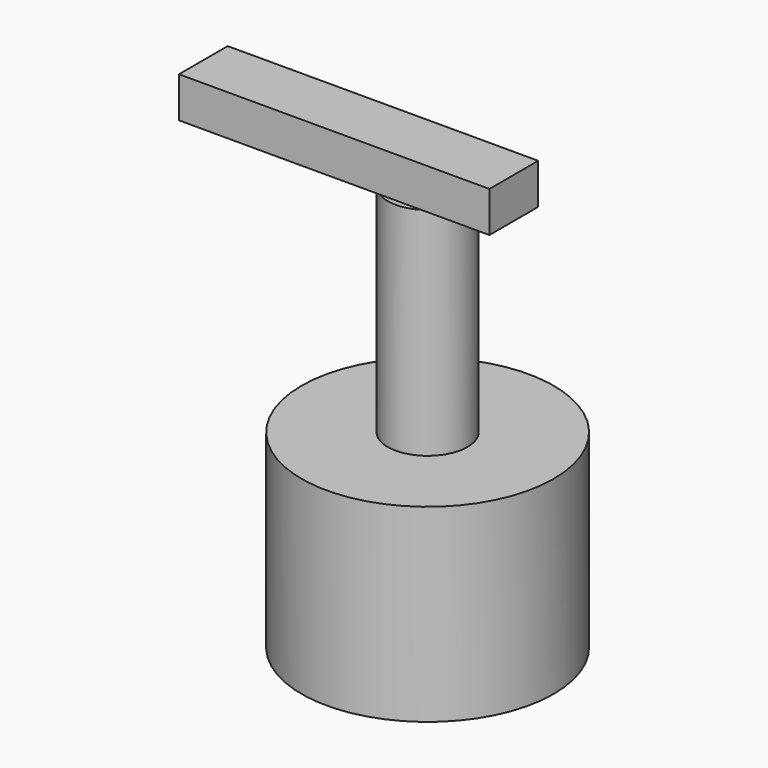
from build123d import *

# Parameters (mm, degrees)
F0_R     = 118.3690263596
F1_DEPTH = 177.8
F2_R     = 37.4516479343
F3_DEPTH = 203.2
F5_DEPTH = 38.1


with BuildPart() as f1:
    # F0 (on Top) → F1 (new body)
    with BuildSketch(Plane.XY):
        Circle(F0_R)
    extrude(amount=F1_DEPTH)

    # F2 (on face) → F3 (join)
    with BuildSketch(Plane.XY.offset(177.8)):
        Circle(F2_R)
    extrude(amount=F3_DEPTH)

    # F4 (on face) → F5 (join)
    with BuildSketch(Plane.XY.offset(381)):
        with BuildLine():
            Line((27.6787410495, 25.2292137593), (0, 25.2292137593))
            Line((0, 25.2292137593), (-27.6787410495, 25.2292137593))
            ThreePointArc((-27.6787410495, 25.2292137593), (-37.0697451311, -5.3347848045), (-19.441274734, -32.0103541017))
            Line((-19.441274734, -32.0103541017), (0, -32.0103541017))
            Line((0, -32.0103541017), (19.441274734, -32.0103541017))
            ThreePointArc((19.441274734, -32.0103541017), (32.6399579483, -18.3646148376), (37.4516479343, 0))
            ThreePointArc((37.4516479343, 0), (34.9230611348, 13.5279611906), (27.6787410495, 25.2292137593))
        make_face()
        with BuildLine():
            Line((83.6336314678, 25.2292137593), (27.6787410495, 25.2292137593))
            ThreePointArc((27.6787410495, 25.2292137593), (34.9230611348, 13.5279611906), (37.4516479343, 0))
            ThreePointArc((37.4516479343, 0), (32.6399579483, -18.3646148376), (19.441274734, -32.0103541017))
            Line((19.441274734, -32.0103541017), (83.6336314678, -32.0103541017))
            Line((83.6336314678, -32.0103541017), (83.6336314678, 0))
            Line((83.6336314678, 0), (83.6336314678, 25.2292137593))
        make_face()
        with BuildLine():
            ThreePointArc((-19.441274734, -32.0103541017), (-37.0697451311, -5.3347848045), (-27.6787410495, 25.2292137593))
            Line((-27.6787410495, 25.2292137593), (-207.8490108252, 25.2292137593))
            Line((-207.8490108252, 25.2292137593), (-207.8490108252, 0))
            Line((-207.8490108252, 0), (-207.8490108252, -32.0103541017))
            Line((-207.8490108252, -32.0103541017), (-19.441274734, -32.0103541017))
        make_face()
    extrude(amount=F5_DEPTH)


solid = f1.part
